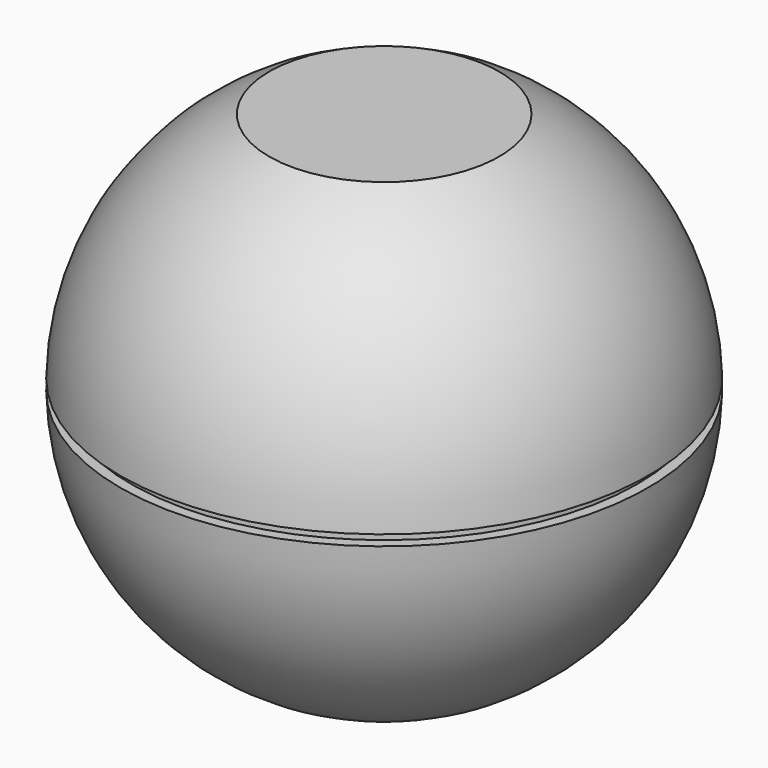
from build123d import *

# Parameters (mm, degrees)
F4_W          = 98.152165938
F4_H          = 19.5652123008
F5_DEPTH      = 25
F5_DEPTH_BACK = 25
F6_W          = 12.6501991157
F6_H          = 2


# Not quite as in the source:
# - a pattern or mirror of a feature is missing from the dataset's text; its kind, count and spacing are read off the source's solid


with BuildPart() as f1:
    # F0 (on Front) → F1 (revolve)
    with BuildSketch(Plane.XZ):
        with BuildLine():
            Line((0, -50), (0, 50))
            ThreePointArc((0, 50), (-50, 0), (0, -50))
        make_face()
    revolve(axis=Axis((0, 0, 0), (0, 0, -1)))

    # F2 (on Front) → F3 (revolve, cut)
    with BuildSketch(Plane.XZ):
        with BuildLine():
            Line((-55, 52.5), (-55, 7.5))
            ThreePointArc((-55, 7.5), (-32.5, 30), (-55, 52.5))
        make_face()
    revolve(axis=Axis((-55, 0, 30), (0, 0, -1)), mode=Mode.SUBTRACT)

    # F4 (on Front) → F5 (cut, two sides)
    with BuildSketch(Plane.XZ) as f5_sk:
        with Locations((0.7781628519, 54.7826061504)):
            Rectangle(F4_W, F4_H)
    f5 = extrude(amount=-F5_DEPTH, mode=Mode.SUBTRACT) + extrude(f5_sk.sketch, amount=F5_DEPTH_BACK, mode=Mode.SUBTRACT)

    # F5_copies: F5 across plane
    add(f5.mirror(Plane(origin=(0, 0, 0), x_dir=(-1, 0, 0), z_dir=(0, 0, -1))), mode=Mode.SUBTRACT)

    # F6 (on Front) → F7 (revolve, cut)
    with BuildSketch(Plane.XZ):
        with Locations((-54.3250995579, -0.0474521765)):
            Rectangle(F6_W, F6_H)
    revolve(axis=Axis((0, 0, 21.1794096977), (0, 0, 1)), mode=Mode.SUBTRACT)


solid = f1.part
